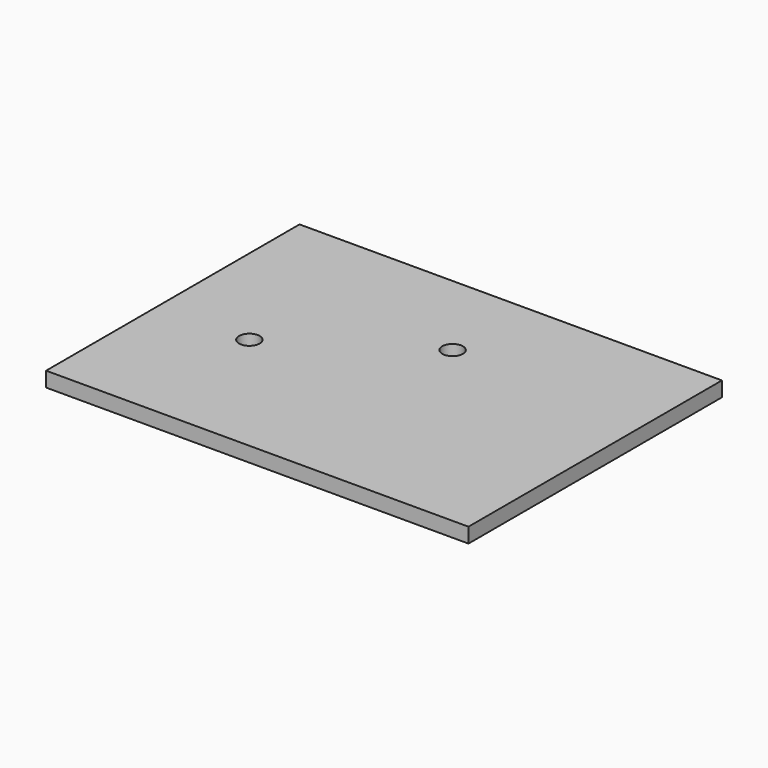
from build123d import *

# Parameters (mm, degrees)
F0_W     = 90
F0_H     = 67.5
F1_DEPTH = 3.175
F3_D     = 4.4


# Not quite as in the source:
# - a length typed as a fraction of an inch, garbled in the dataset ("3 / 203.2 mm" for 3/8 in), is restored


with BuildPart() as f1:
    # F0 (on Top) → F1 (new body)
    with BuildSketch(Plane.XY):
        Rectangle(F0_W, F0_H)
    extrude(amount=F1_DEPTH)

    # F3 (through all)
    with Locations(Plane.XY.offset(3.175)):
        with Locations((-25.553, -3.925), (3.175, 14.303)):
            Hole(F3_D / 2)


solid = f1.part
